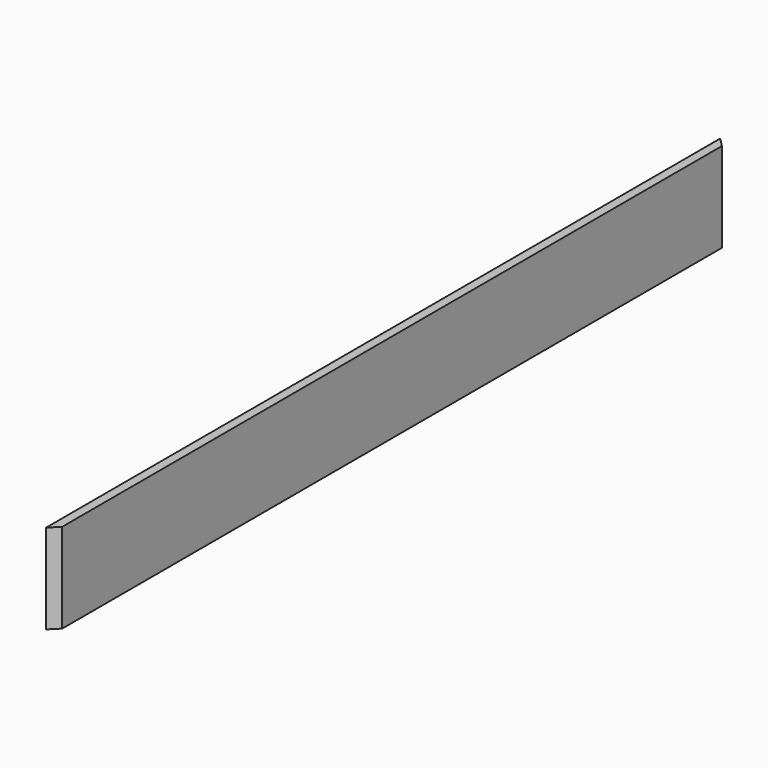
from build123d import *

# Parameters (mm, degrees)
F0_W        = 19.05
F0_H        = 190.5
F1_DEPTH    = 914.4
F2_T1_DEPTH = 386.462243683


# Not quite as in the source:
# - a fillet or chamfer that OpenCascade refuses, or shapes differently, is made with other operations: its cross-section is extruded or revolved along the edge and cut away or added


with BuildPart() as f1:
    # F0 (on Front) → F1 (new body, symmetric)
    with BuildSketch(Plane.XZ):
        Rectangle(F0_W, F0_H)
    extrude(amount=F1_DEPTH, both=True)

    # F2: chamfer of 38.1 on 2 edges, made by hand

    # F2_s2 → F2_t1 (cut)
    with BuildSketch(Plane.XY.offset(-193.2311218415)):
        Polygon((9.525, -876.3), (-28.575, -914.4), (9.525, -914.4), align=None)
        Polygon((9.525, 876.3), (-28.575, 914.4), (9.525, 914.4), align=None)
    extrude(amount=F2_T1_DEPTH, mode=Mode.SUBTRACT)


solid = f1.part
